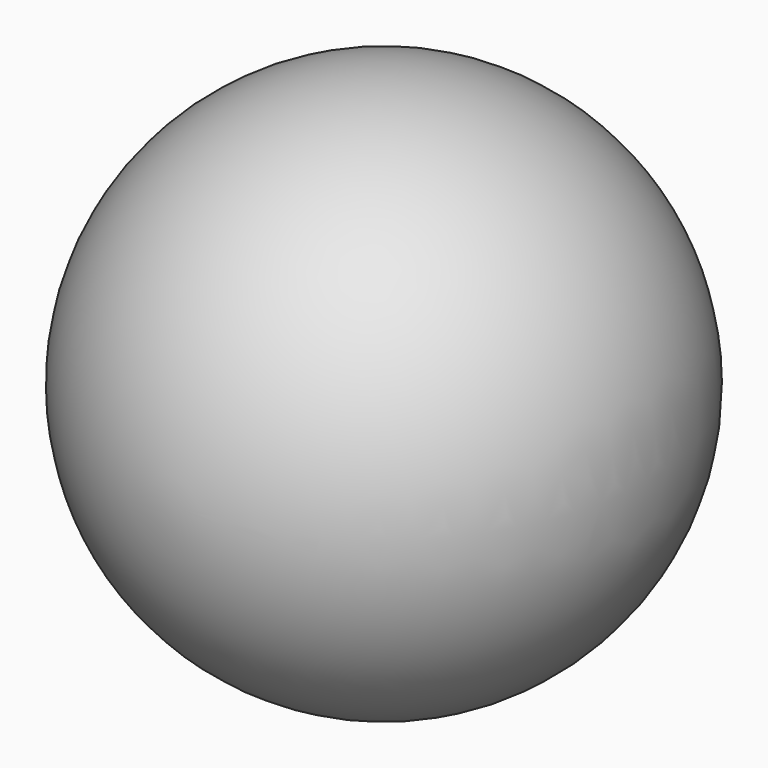
from build123d import *

# Parameters (mm, degrees)
F6_W     = 6.0810809955
F6_H     = 35.6756746769
F7_DEPTH = 39.5


# Not quite as in the source:
# - the program builds the solid bodies; features that only make, move or delete a surface that nothing else refers to are left out


with BuildPart() as f5:
    # F4 (on Top) → F5 (revolve)
    with BuildSketch(Plane.XY):
        with BuildLine():
            Line((0, 73.5685819782), (0, 49.8039578997))
            ThreePointArc((0, 49.8039578997), (11.8823120393, 61.6862699389), (0, 73.5685819782))
        make_face()
    revolve(axis=Axis((0, 10.8100157231, 0), (0, -1, 0)))

    # F6 (on Right) → F7 (cut, symmetric)
    with BuildSketch(Plane.YZ):
        with Locations((14.0385185368, 40.8424846828)):
            Rectangle(F6_W, F6_H)
    extrude(amount=F7_DEPTH, both=True, mode=Mode.SUBTRACT)


solid = f5.part
